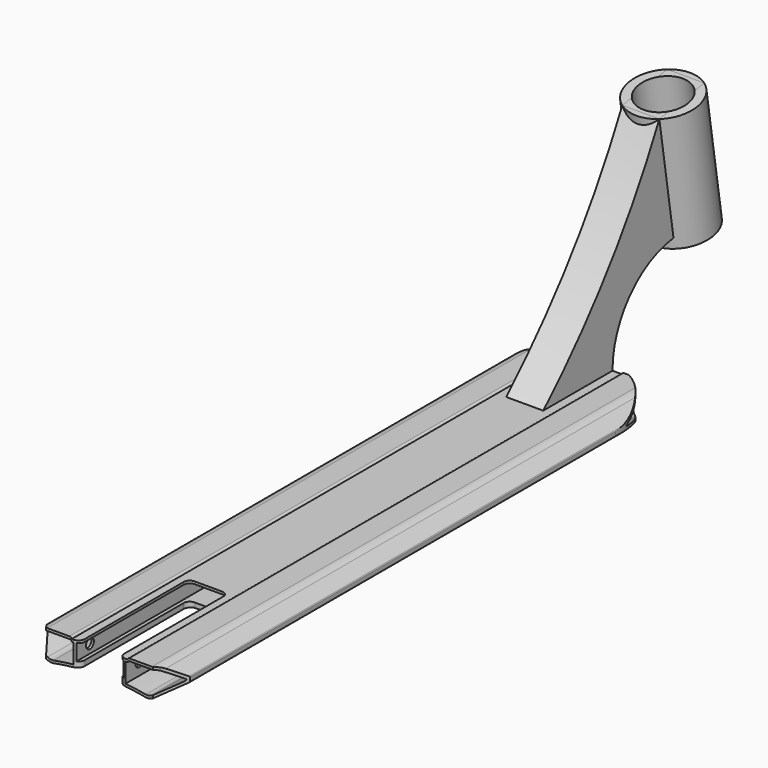
from build123d import *

# Parameters (mm, degrees)
F1_DEPTH       = 250
F2_W           = 38
F2_H           = 13
F3_DEPTH       = 250
F4_T1_DEPTH    = 509.3674969976
F5_R           = 9
F6_R           = 1
F8_DEPTH       = 500.001
F10_DEPTH      = 24.4523840141
F10_DEPTH_BACK = 527
F12_DEPTH      = 527
F12_DEPTH_BACK = 24.4523841141
F13_F1_R       = 4.9999
F13_F2_R       = 4.9999
F13_F3_R       = 5
F13_F4_R       = 5
F13_F5_R       = 5
F13_F6_R       = 5
F15_DEPTH      = 15
F16_R          = 27.4590604355
F17_DEPTH      = 100
F19_D          = 40
F21_D          = 8
F21_DEPTH      = 50
F21_TIP        = 2.4034424761


# Not quite as in the source:
# - a fillet or chamfer that OpenCascade refuses, or shapes differently, is made with other operations: its cross-section is extruded or revolved along the edge and cut away or added
# - a fillet or chamfer is up to 0.001 mm smaller than in the source, because OpenCascade refuses the exact size
# - an extrude ends at something that could not be found from the text; its depth is read off the source's solid


with BuildPart() as f1:
    # F0 (on Front) → F1 (new body, symmetric)
    with BuildSketch(Plane.XZ):
        with BuildLine():
            Line((22.5, 23.1513840141), (0, 23.1513840141))
            Line((0, 23.1513840141), (-22.5, 23.1513840141))
            Line((-22.5, 23.1513840141), (-22.5, 24.4513840141))
            Line((-22.5, 24.4513840141), (-45.5824640741, 24.4513840141))
            Line((-45.5824640741, 24.4513840141), (-57.5, 14.4513840141))
            Line((-57.5, 14.4513840141), (-57.5, 10.4513840141))
            Line((-57.5, 10.4513840141), (-40.1794919243, 0.4513840141))
            ThreePointArc((-40.1794919243, 0.4513840141), (0, 4.5289288725), (40.1794919243, 0.4513840141))
            Line((40.1794919243, 0.4513840141), (57.5, 10.4513840141))
            Line((57.5, 10.4513840141), (57.5, 14.4513840141))
            Line((57.5, 14.4513840141), (45.5824640741, 24.4513840141))
            Line((45.5824640741, 24.4513840141), (22.5, 24.4513840141))
            Line((22.5, 24.4513840141), (22.5, 23.1513840141))
        make_face()
    extrude(amount=F1_DEPTH, both=True)

    # F2 (on Front) → F3 (cut, symmetric)
    with BuildSketch(Plane.XZ):
        with Locations((0, 14.6513840141)):
            Rectangle(F2_W, F2_H)
    extrude(amount=F3_DEPTH, both=True, mode=Mode.SUBTRACT)

    # F4: fillet of radius 2 on 2 edges, made by hand

    # F4_s2 → F4_t1 (cut)
    with BuildSketch(Plane.XZ.offset(-254.6837484988)):
        with BuildLine():
            ThreePointArc((-24.3734993995, 24.4513840141), (-23.2333239744, 24.0945516866), (-22.5, 23.1513840141))
            Line((-22.5, 23.1513840141), (-22.5, 24.4513840141))
            Line((-22.5, 24.4513840141), (-24.3734993995, 24.4513840141))
        make_face()
        with BuildLine():
            ThreePointArc((24.3734993995, 24.4513840141), (23.2333239744, 24.0945516866), (22.5, 23.1513840141))
            Line((22.5, 23.1513840141), (22.5, 24.4513840141))
            Line((22.5, 24.4513840141), (24.3734993995, 24.4513840141))
        make_face()
    extrude(amount=F4_T1_DEPTH, mode=Mode.SUBTRACT)

    # F5
    f5_edges = [f1.edges().sort_by_distance(p)[0] for p in [
        (-45.582464, 0, 24.451384),
        (-40.179492, 0, 0.451384),
        (40.179492, 0, 0.451384),
        (45.582464, 0, 24.451384),
    ]]
    fillet(f5_edges, radius=F5_R)

    # F6
    f6_edges = [f1.edges().sort_by_distance(p)[0] for p in [
        (57.5, 0, 14.451384),
        (57.5, 0, 10.451384),
        (-57.5, 0, 10.451384),
        (-57.5, 0, 14.451384),
    ]]
    fillet(f6_edges, radius=F6_R)

    # F7 (on face) → F8 (cut, through all)
    with BuildSketch(Plane.XZ.offset(250)):
        with BuildLine():
            ThreePointArc((-42.1022690923, 3.8709010064), (-39.7790673433, 3.0327059534), (-37.3093701274, 3.0535140017))
            ThreePointArc((-37.3093701274, 3.0535140017), (-29.1789785809, 4.4103617496), (-21, 5.4343792715))
            Line((-21, 5.4343792715), (-21, 21.1513840141))
            Line((-21, 21.1513840141), (-22.5, 21.1513840141))
            ThreePointArc((-22.5, 21.1513840141), (-23.2333239744, 22.0945516866), (-24.3734993995, 22.4513840141))
            Line((-24.3734993995, 22.4513840141), (-42.3067319657, 22.4513840141))
            ThreePointArc((-42.3067319657, 22.4513840141), (-44.7008729689, 22.0292323596), (-46.8062452335, 20.813695116))
            Line((-46.8062452335, 20.813695116), (-55.7563117574, 13.3036975967))
            ThreePointArc((-55.7563117574, 13.3036975967), (-56.1097188459, 12.4504974108), (-55.6135241478, 11.6716277498))
            Line((-55.6135241478, 11.6716277498), (-42.1022690923, 3.8709010064))
        make_face()
        with BuildLine():
            Line((21, 21.1513840141), (21, 5.4343792715))
            ThreePointArc((21, 5.4343792715), (29.1789785809, 4.4103617496), (37.3093701274, 3.0535140017))
            ThreePointArc((37.3093701274, 3.0535140017), (39.7790673433, 3.0327059534), (42.1022690923, 3.8709010064))
            Line((42.1022690923, 3.8709010064), (55.6135241478, 11.6716277498))
            ThreePointArc((55.6135241478, 11.6716277498), (56.1097188459, 12.4504974108), (55.7563117574, 13.3036975967))
            Line((55.7563117574, 13.3036975967), (46.8062452335, 20.813695116))
            ThreePointArc((46.8062452335, 20.813695116), (44.7008729689, 22.0292323596), (42.3067319657, 22.4513840141))
            Line((42.3067319657, 22.4513840141), (24.3734993995, 22.4513840141))
            ThreePointArc((24.3734993995, 22.4513840141), (23.2333239744, 22.0945516866), (22.5, 21.1513840141))
            Line((22.5, 21.1513840141), (21, 21.1513840141))
        make_face()
    extrude(amount=-F8_DEPTH, mode=Mode.SUBTRACT)

    # F9 (on Top) → F10 (cut, two sides)
    with BuildSketch(Plane.XY) as f10_sk:
        with BuildLine():
            ThreePointArc((-57.5, 200), (0, 257.5), (57.5, 200))
            Line((57.5, 200), (57.5, 280))
            Line((57.5, 280), (-57.5, 280))
            Line((-57.5, 280), (-57.5, 200))
        make_face()
    extrude(amount=F10_DEPTH, mode=Mode.SUBTRACT)
    extrude(f10_sk.sketch, amount=-F10_DEPTH_BACK, mode=Mode.SUBTRACT)

    # F11 (on Top) → F12 (cut, two sides)
    with BuildSketch(Plane.XY) as f12_sk:
        Polygon((-43.2975540478, -250), (-68, -216), (-68, -346), (68, -346), (68, -216), (43.2975540478, -250), (16, -250), (16, -140), (-16, -140), (-16, -250), align=None)
    extrude(amount=-F12_DEPTH, mode=Mode.SUBTRACT)
    extrude(f12_sk.sketch, amount=F12_DEPTH_BACK, mode=Mode.SUBTRACT)

    # F13: fillet of radius 5 on 8 edges, made by hand

    # F13_f1 (radius 5 in the source; OpenCascade refuses exactly that, so slightly less here)
    f13_f1_edges = [f1.edges().sort_by_distance(p)[0] for p in [
        (-16, -250, 22.1513840141),
    ]]
    fillet(f13_f1_edges, radius=F13_F1_R)

    # F13_f2 (radius 5 in the source; OpenCascade refuses exactly that, so slightly less here)
    f13_f2_edges = [f1.edges().sort_by_distance(p)[0] for p in [
        (16, -250, 6.0196427984),
    ]]
    fillet(f13_f2_edges, radius=F13_F2_R)

    # F13_f3
    f13_f3_edges = [f1.edges().sort_by_distance(p)[0] for p in [
        (16, -140, 22.1513840141),
    ]]
    fillet(f13_f3_edges, radius=F13_F3_R)

    # F13_f4
    f13_f4_edges = [f1.edges().sort_by_distance(p)[0] for p in [
        (-16, -140, 22.1513840141),
    ]]
    fillet(f13_f4_edges, radius=F13_F4_R)

    # F13_f5
    f13_f5_edges = [f1.edges().sort_by_distance(p)[0] for p in [
        (-16, -140, 6.0196427984),
    ]]
    fillet(f13_f5_edges, radius=F13_F5_R)

    # F13_f6
    f13_f6_edges = [f1.edges().sort_by_distance(p)[0] for p in [
        (16, -140, 6.0196427984),
    ]]
    fillet(f13_f6_edges, radius=F13_F6_R)

    # F14 (on Right) → F15 (join, symmetric)
    with BuildSketch(Plane.YZ):
        with BuildLine():
            ThreePointArc((297.3819995028, 183.1513840141), (245.9666940414, 97.8136618671), (180, 23.1513840141))
            Line((180, 23.1513840141), (250, 23.1513840141))
            ThreePointArc((250, 23.1513840141), (267.6550746197, 69.6272787008), (311.7145367693, 92.6593051387))
            Line((311.7145367693, 92.6593051387), (313.0254460068, 84.3825499546))
            Line((313.0254460068, 84.3825499546), (358.4591096742, 91.5785353465))
            Line((358.4591096742, 91.5785353465), (342.8156631702, 190.347369406))
            Line((342.8156631702, 190.347369406), (297.3819995028, 183.1513840141))
        make_face()
    extrude(amount=F15_DEPTH, both=True)

    # F16 (on face) → F17 (join, through all)
    with BuildSketch(Plane(origin=(0, -21.0209895784, 132.7213047908), x_dir=(1, 0, 0), z_dir=(0, -0.156434465, 0.9876883406))):
        with Locations((0, 345.3719223914)):
            Circle(F16_R)
    extrude(amount=-F17_DEPTH)

    # F19 (through all)
    with Locations(Plane(origin=(0, -21.0209895784, 132.7213047908), x_dir=(1, 0, 0), z_dir=(0, -0.156434465, 0.9876883406))):
        with Locations((0, 345.3719223914)):
            Hole(F19_D / 2)

    # F21 (one way)
    with BuildSketch(Plane.YZ.offset(21)):
        with Locations((-236, 15.4343792715)):
            Circle(F21_D / 2)
    extrude(amount=-F21_DEPTH, mode=Mode.SUBTRACT)
    with Locations(Plane.YZ.offset(21)):
        with Locations((-236, 15.4343792715)):
            with Locations((0, 0, -(F21_DEPTH + F21_TIP / 2))):  # 118° drill point
                Cone(0, F21_D / 2, F21_TIP, mode=Mode.SUBTRACT)


solid = f1.part
